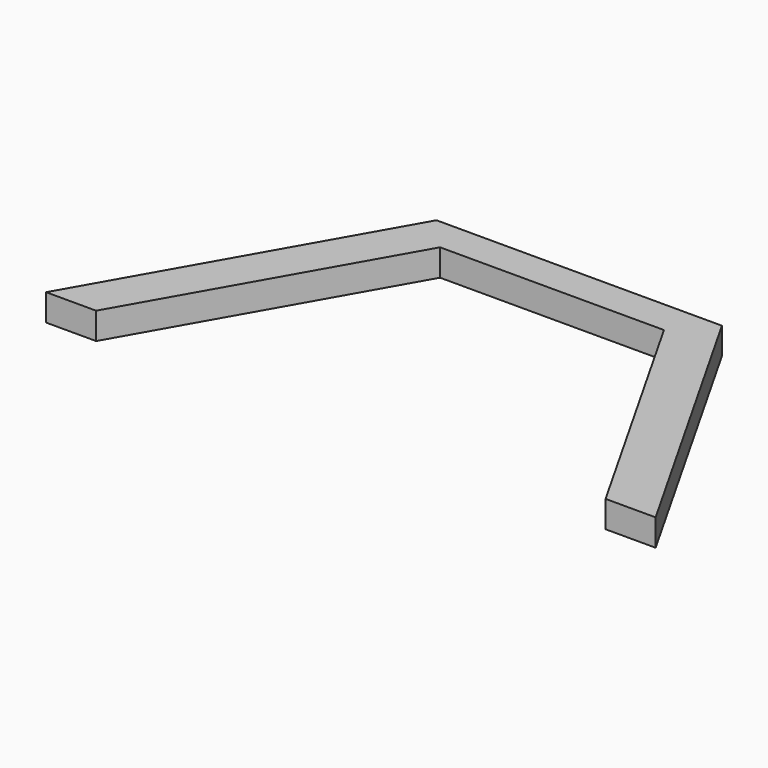
from build123d import *

# Parameters (mm, degrees)
F1_DEPTH = 9.525


# Not quite as in the source:
# - a length typed as a fraction of an inch, garbled in the dataset ("3 / 203.2 mm" for 3/8 in), is restored
# - a feature names something its author has since deleted; it is built from what else it names


with BuildPart() as f1:
    # F0 (on Top) → F1 (new body)
    with BuildSketch(Plane.XY):
        Polygon((44.3405605153, 56.6629169657), (-6.4594394847, 56.6629169657), (-57.2594394847, 56.6629169657), (-114.934632644, -44.9370830343), (-97.1201658249, -44.9370830343), (-46.3125111366, 44.5651350522), (-6.4594394847, 44.5651350522), (33.3936321673, 44.5651350522), (84.2012868556, -44.9370830343), (102.0157536747, -44.9370830343), align=None)
    extrude(amount=F1_DEPTH)


solid = f1.part
